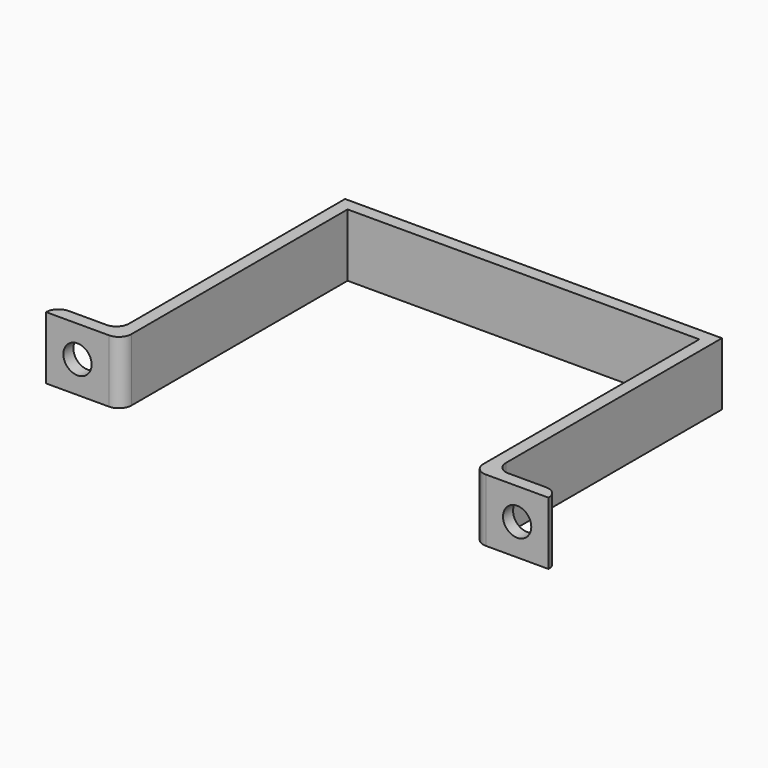
from build123d import *

# Parameters (mm, degrees)
F1_DEPTH = 5
F3_D     = 4.4958
F4_R     = 1.99999


# Not quite as in the source:
# - a fillet or chamfer is up to 0.001 mm smaller than in the source, because OpenCascade refuses the exact size


with BuildPart() as f1:
    # F0 (on Top) → F1 (new body, symmetric)
    with BuildSketch(Plane.XY):
        Polygon((0, 47), (0, 45), (28, 45), (28, 0), (40, 0), (40, 2), (30, 2), (30, 47), align=None)
    extrude(amount=F1_DEPTH, both=True)

    # F3 (through all)
    with Locations(Plane(origin=(0, 2, 0), x_dir=(-1, 0, 0), z_dir=(0, 1, 0))):
        with Locations((-35, 0)):
            Hole(F3_D / 2)

    # F4 (radius 2 in the source; OpenCascade refuses exactly that, so slightly less here)
    f4_edges = [f1.edges().sort_by_distance(p)[0] for p in [
        (30, 2, 0),
        (28, 0, 0),
        (40, 2, 0),
    ]]
    fillet(f4_edges, radius=F4_R)

    # F5: F1 across plane


with BuildPart() as f1_1:
    add(f1.part)
    add(f1.part.mirror(Plane.YZ))


solid = f1_1.part
